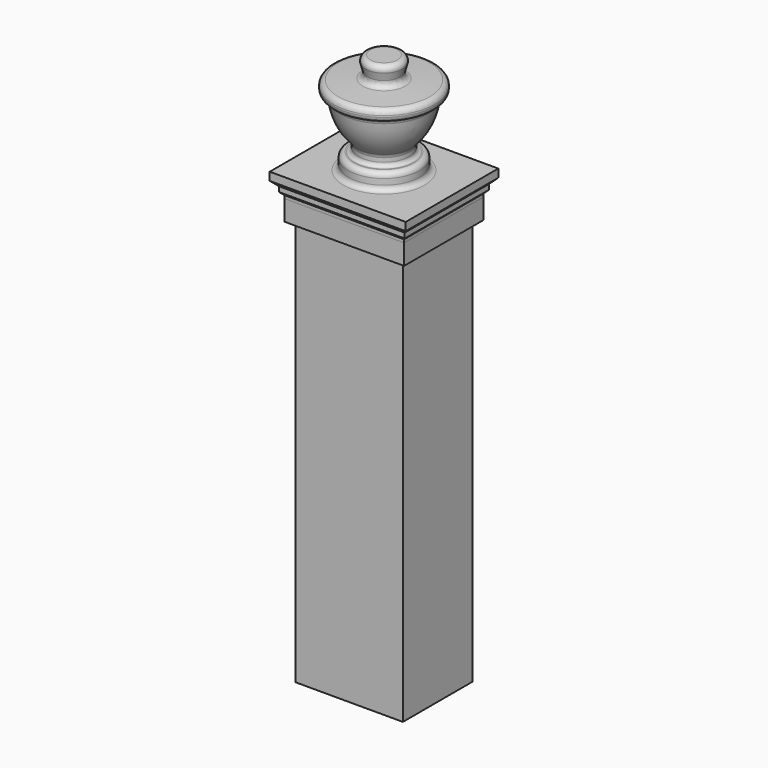
from build123d import *

# Parameters (mm, degrees)
F0_W     = 530
F0_H     = 430
F1_DEPTH = 2000
F2_W     = 590
F2_H     = 490
F3_DEPTH = 100
F6_W     = 510
F6_H     = 410
F7_DEPTH = 120
F10_R    = 25.4
F11_R    = 19.05


with BuildPart() as f1:
    # F0 (on Top) → F1 (new body)
    with BuildSketch(Plane.XY):
        Rectangle(F0_W, F0_H)
    extrude(amount=F1_DEPTH)

    # F2 (on face) → F3 (join)
    with BuildSketch(Plane.XY.offset(2000)):
        Rectangle(F2_W, F2_H)
    extrude(amount=F3_DEPTH)


with BuildPart() as f5:
    # F5: sweep along a path in F5_path
    with BuildLine(Plane(origin=(295, -245, 2100), x_dir=(0, 1, 0), z_dir=(0, 0, 1))) as f5_path:
        Line((0, 0), (0, 590))
        Line((0, 590), (490, 590))
        Line((490, 590), (490, 0))
        Line((490, 0), (0, 0))
    # F4 (on Right) → F5 (sweep)
    with BuildSketch(Plane.YZ):
        Polygon((-245, 2115), (-245, 2100), (-205, 2100), (-205, 2220), (-285, 2220), (-285, 2180), (-260, 2155), (-260, 2130), align=None)
    sweep(path=f5_path.line, transition=Transition.RIGHT)

    # F6 (on face) → F7 (join, through all)
    with BuildSketch(Plane.XY.offset(2220)):
        Rectangle(F6_W, F6_H)
    extrude(amount=-F7_DEPTH)

    # F8 (on Right) → F9 (revolve)
    with BuildSketch(Plane.YZ):
        with BuildLine():
            Line((100, 2720), (0, 2720))
            Line((0, 2720), (0, 2220))
            Line((0, 2220), (175, 2220))
            Line((175, 2220), (175, 2300))
            Line((175, 2300), (125, 2300))
            Line((125, 2300), (125, 2349.1206169128))
            ThreePointArc((125, 2349.1206169128), (189.7823627721, 2440.179500918), (216.7436426898, 2548.6302467329))
            Line((216.7436426898, 2548.6302467329), (250, 2560.7345708939))
            Line((250, 2560.7345708939), (250, 2610.7345708939))
            Line((250, 2610.7345708939), (73.2050807569, 2620))
            Line((73.2050807569, 2620), (100, 2720))
        make_face()
    revolve(axis=Axis((0, 0, 1360), (0, 0, 1)))

    # F10
    f10_edges = [f5.edges().sort_by_distance(p)[0] for p in [
        (0, -175, 2220),
        (0, -175, 2300),
        (0, -125, 2349.120617),
        (0, -216.743643, 2548.630247),
        (0, -73.205081, 2620),
        (0, -250, 2560.734571),
        (0, -250, 2610.734571),
        (0, -100, 2720),
    ]]
    fillet(f10_edges, radius=F10_R)

    # F11
    f11_edges = [f5.edges().sort_by_distance(p)[0] for p in [
        (0, -125, 2300),
    ]]
    fillet(f11_edges, radius=F11_R)


solid = Compound([f1.part, f5.part])
